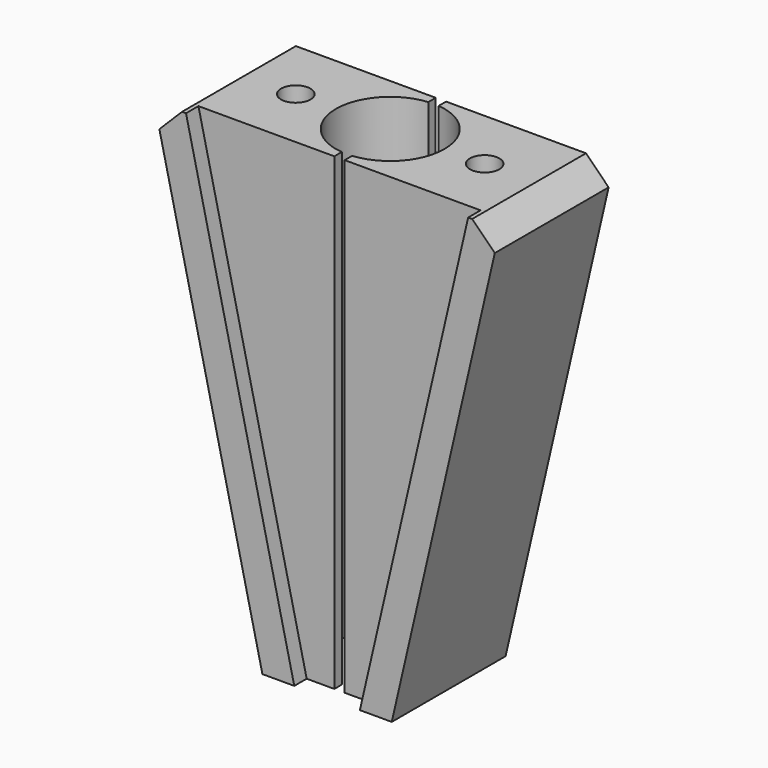
from build123d import *

# Parameters (mm, degrees)
F1_DEPTH = 27.94
F3_DEPTH = 3.048
F5_D     = 5.7912
F5_DEPTH = 22.86
F5_TIP   = 1.7398520085
F7_D     = 21.336
F8_W     = 2.032
F8_H     = 92.075
F9_DEPTH = 24.893


# Not quite as in the source:
# - a feature names something its author has since deleted; it is built from what else it names


with BuildPart() as f1:
    # F0 (on Front) → F1 (new body)
    with BuildSketch(Plane.XZ):
        Polygon((12.7, -92.075), (32.9309795883, -4.445), (28.4859795883, 0), (-28.4859795883, 0), (-32.9309795883, -4.445), (-12.7, -92.075), align=None)
    extrude(amount=-F1_DEPTH)

    # F2 (on face) → F3 (cut)
    with BuildSketch(Plane.XZ):
        Polygon((-27.7008388568, 0), (-6.4436501589, -92.075), (6.4436501589, -92.075), (27.7008388568, 0), align=None)
    extrude(amount=-F3_DEPTH, mode=Mode.SUBTRACT)

    # F5
    with Locations(Plane.XY):
        with Locations((-18.542, 15.494), (18.542, 15.494)):
            Hole(F5_D / 2, depth=F5_DEPTH)
            with Locations((0, 0, -(F5_DEPTH + F5_TIP / 2))):  # 118° drill point
                Cone(0, F5_D / 2, F5_TIP, mode=Mode.SUBTRACT)

    # F7 (through all)
    with Locations(Plane.XY):
        with Locations((0, 15.494)):
            Hole(F7_D / 2)

    # F8 (on face) → F9 (cut, through all)
    with BuildSketch(Plane.XZ.offset(-3.048)):
        with Locations((0, -46.0375)):
            Rectangle(F8_W, F8_H)
    extrude(amount=-F9_DEPTH, mode=Mode.SUBTRACT)


solid = f1.part
